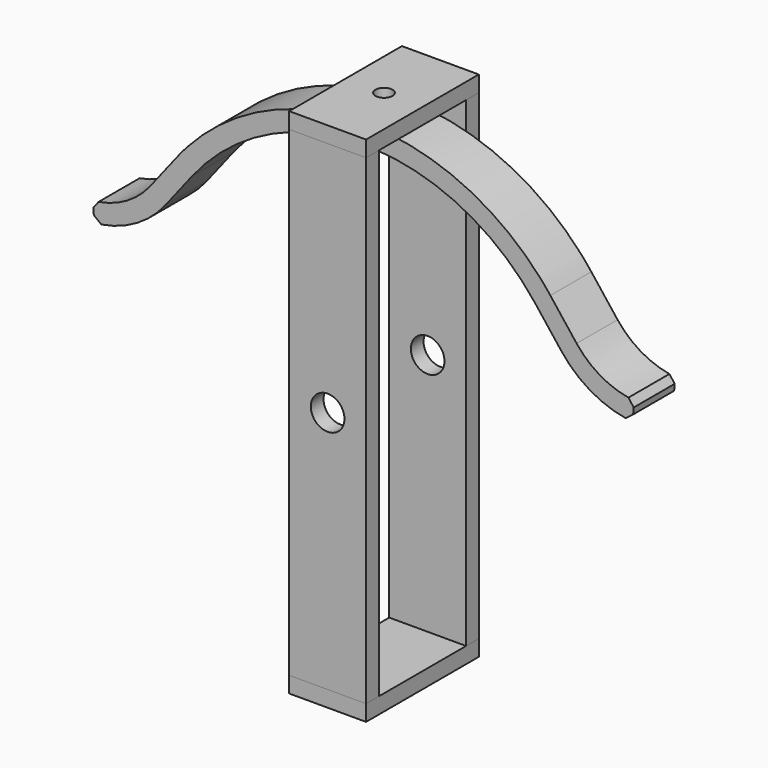
from build123d import *

# Parameters (mm, degrees)
F1_DEPTH    = 12.7
F2_T1_DEPTH = 41.1780168926
F2_T3_DEPTH = 42.797567125
F3_W        = 38.1
F3_H        = 7.9502
F4_DEPTH    = 34.925
F5_W        = 38.1
F5_H        = 7.874
F6_DEPTH    = 238.252
F8_D        = 16.6624
F8_2_D      = 16.6624
F10_D       = 5.1054
F10_DEPTH   = 12.7
F10_TIP     = 1.5338169022
F10_2_D     = 5.1054
F10_2_DEPTH = 12.7
F10_2_TIP   = 1.5338169022
F12_D       = 8.4328
F12_DEPTH   = 27.305
F12_TIP     = 2.5334687141
F13_W       = 38.1
F13_H       = 69.85
F13_R       = 2.5527
F14_DEPTH   = 7.9502


# Not quite as in the source:
# - a fillet or chamfer that OpenCascade refuses, or shapes differently, is made with other operations: its cross-section is extruded or revolved along the edge and cut away or added


with BuildPart() as f1:
    # F0 (on Front) → F1 (new body, symmetric)
    with BuildSketch(Plane.XZ):
        with BuildLine():
            Line((-134.254875, 39.8868755789), (-133.35, 30.4049545586))
            ThreePointArc((-133.35, 30.4049545586), (-113.74755339, 36.4343087177), (-98.1266094704, 49.7232189715))
            Line((-98.1266094704, 49.7232189715), (-85.1049548754, 66.4104596856))
            ThreePointArc((-85.1049548754, 66.4104596856), (0, 107.95), (85.1049548754, 66.4104596856))
            Line((85.1049548754, 66.4104596856), (98.1266094704, 49.7232189715))
            ThreePointArc((98.1266094704, 49.7232189715), (113.74755339, 36.4343087177), (133.35, 30.4049545586))
            Line((133.35, 30.4049545586), (134.254875, 39.8868755789))
            ThreePointArc((134.254875, 39.8868755789), (118.3278871294, 44.7857258331), (105.6358701947, 55.5829654143))
            Line((105.6358701947, 55.5829654143), (92.6142155997, 72.2702061284))
            ThreePointArc((92.6142155997, 72.2702061284), (90.0794962204, 75.4059678386), (87.4386569195, 78.4528960658))
            ThreePointArc((87.4386569195, 78.4528960658), (0, 117.475), (-87.4386569195, 78.4528960658))
            ThreePointArc((-87.4386569195, 78.4528960658), (-90.0794962204, 75.4059678386), (-92.6142155997, 72.2702061284))
            Line((-92.6142155997, 72.2702061284), (-105.6358701947, 55.5829654143))
            ThreePointArc((-105.6358701947, 55.5829654143), (-118.3278871294, 44.7857258331), (-134.254875, 39.8868755789))
        make_face()
    extrude(amount=F1_DEPTH, both=True)

    # F2: chamfer of 3.175 on 4 edges, made by hand

    # F2_s2 → F2_t1 (cut)
    with BuildSketch(Plane.XZ.offset(-20.5890084463)):
        with BuildLine():
            Line((131.3300103455, 40.2719071277), (133.9640360968, 36.839259599))
            Line((133.9640360968, 36.839259599), (134.254875, 39.8868755789))
            ThreePointArc((134.254875, 39.8868755789), (132.7444106107, 40.0591461616), (131.3300103455, 40.2719071277))
        make_face()
        with BuildLine():
            Line((-133.9640360968, 36.839259599), (-131.3300103455, 40.2719071277))
            ThreePointArc((-131.3300103455, 40.2719071277), (-132.7444106107, 40.0591461616), (-134.254875, 39.8868755789))
            Line((-134.254875, 39.8868755789), (-133.9640360968, 36.839259599))
        make_face()
    extrude(amount=F2_T1_DEPTH, mode=Mode.SUBTRACT)

    # F2_s4 → F2_t3 (cut)
    with BuildSketch(Plane.XZ.offset(-21.3987835625)):
        with BuildLine():
            Line((133.6616903629, 33.6710668983), (129.989386691, 30.8391913582))
            ThreePointArc((129.989386691, 30.8391913582), (131.6215577531, 30.5998162612), (133.35, 30.4049545586))
            Line((133.35, 30.4049545586), (133.6616903629, 33.6710668983))
        make_face()
        with BuildLine():
            Line((-129.989386691, 30.8391913582), (-133.6616903629, 33.6710668983))
            Line((-133.6616903629, 33.6710668983), (-133.35, 30.4049545586))
            ThreePointArc((-133.35, 30.4049545586), (-131.6215577531, 30.5998162612), (-129.989386691, 30.8391913582))
        make_face()
    extrude(amount=F2_T3_DEPTH, mode=Mode.SUBTRACT)

    # F3 (on Front) → F4 (join, symmetric)
    with BuildSketch(Plane.XZ):
        with Locations((0, 121.44375)):
            Rectangle(F3_W, F3_H)
    extrude(amount=F4_DEPTH, both=True)

    # F12
    with Locations(Plane.XY.offset(125.41885)):
        with Locations((0, 0)):
            Hole(F12_D / 2, depth=F12_DEPTH)
            with Locations((0, 0, -(F12_DEPTH + F12_TIP / 2))):  # 118° drill point
                Cone(0, F12_D / 2, F12_TIP, mode=Mode.SUBTRACT)


with BuildPart() as f6:
    # F5 (on face) → F6 (new body)
    with BuildSketch(Plane(origin=(0, 0, 117.46865), x_dir=(1, 0, 0), z_dir=(0, 0, -1))):
        with Locations((0, 30.988)):
            Rectangle(F5_W, F5_H)
    extrude(amount=F6_DEPTH)

    # F8 (through all)
    with Locations(Plane.XZ.offset(34.925)):
        with Locations((0, 0)):
            Hole(F8_D / 2)

    # F10
    with Locations(Plane(origin=(0, 0, -120.78335), x_dir=(1, 0, 0), z_dir=(0, 0, -1))):
        with Locations((0, 30.988), (0, -30.988)):
            Hole(F10_D / 2, depth=F10_DEPTH)
            with Locations((0, 0, -(F10_DEPTH + F10_TIP / 2))):  # 118° drill point
                Cone(0, F10_D / 2, F10_TIP, mode=Mode.SUBTRACT)


with BuildPart() as f6b:
    # F5 (on face) → F6, piece 2 (new body)
    with BuildSketch(Plane(origin=(0, 0, 117.46865), x_dir=(1, 0, 0), z_dir=(0, 0, -1))):
        with Locations((0, -30.988)):
            Rectangle(F5_W, F5_H)
    extrude(amount=F6_DEPTH)

    # F8#2 (through all)
    with Locations(Plane.XZ.offset(34.925)):
        with Locations((0, 0)):
            Hole(F8_2_D / 2)

    # F10#2
    with Locations(Plane(origin=(0, 0, -120.78335), x_dir=(1, 0, 0), z_dir=(0, 0, -1))):
        with Locations((0, 30.988), (0, -30.988)):
            Hole(F10_2_D / 2, depth=F10_2_DEPTH)
            with Locations((0, 0, -(F10_2_DEPTH + F10_2_TIP / 2))):  # 118° drill point
                Cone(0, F10_2_D / 2, F10_2_TIP, mode=Mode.SUBTRACT)


with BuildPart() as f14:
    # F13 (on face) → F14 (new body)
    with BuildSketch(Plane(origin=(0, 0, -120.78335), x_dir=(1, 0, 0), z_dir=(0, 0, -1))):
        Rectangle(F13_W, F13_H)
        with Locations((0, -30.988)):
            Circle(F13_R, mode=Mode.SUBTRACT)
        with Locations((0, 30.988)):
            Circle(F13_R, mode=Mode.SUBTRACT)
    extrude(amount=F14_DEPTH)


solid = Compound([f1.part, f6.part, f6b.part, f14.part])
